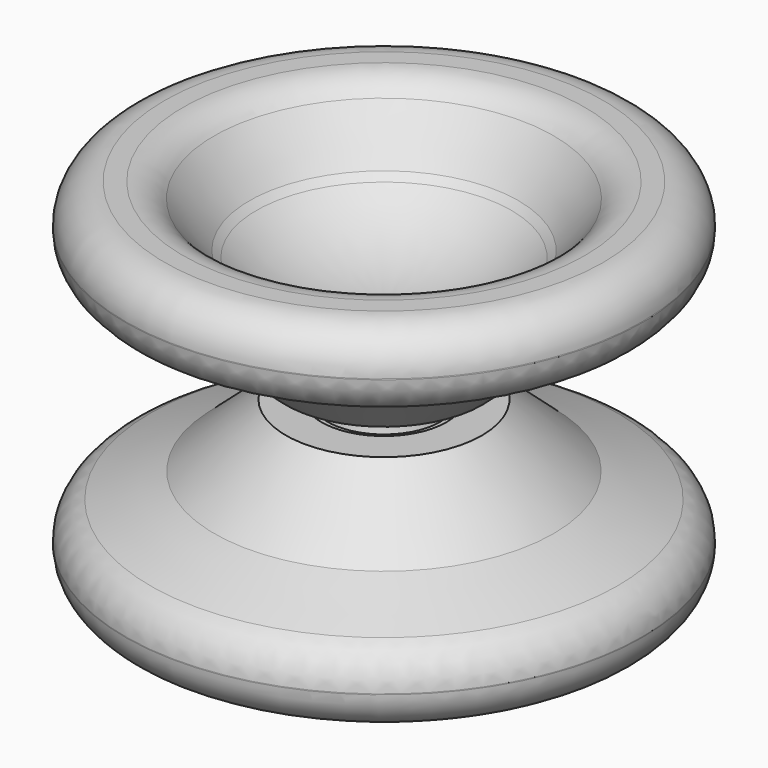
from build123d import *

# Parameters (mm, degrees)
F2_R            = 4.4
F3_R            = 20
F4_W            = 0.825
F4_H            = 3.6
F6_COPIES_COUNT = 10
F8_DEPTH        = 1.7
F8_COPIES_COUNT = 10


# Not quite as in the source:
# - a pattern or mirror of a feature is missing from the dataset's text; its kind, count and spacing are read off the source's solid


with BuildPart() as f1:
    # F0 (on Front) → F1 (revolve)
    with BuildSketch(Plane.XZ):
        Polygon((3.125, 0), (0, 0), (0, -7.5), (8.6189414508, -7.5), (15.0811627811, -13.2031436252), (20.3810585492, -20), (29, -20), (29, -12.5), (19.0302016061, -8.5869428264), (11, -1.5), (7, -1.5), (7, -2), (3.125, -2), align=None)
    revolve(axis=Axis((0, 0, -3.75), (0, 0, -1)))

    # F1_copies: F1 across plane


with BuildPart() as f1_1:
    add(f1.part)
    add(f1.part.mirror(Plane.XY))

    # F2
    f2_edges = [f1_1.edges().sort_by_distance(p)[0] for p in [
        (-29, 0, -12.5),
        (-29, 0, -20),
        (-20.381059, 0, -20),
        (-29, 0, 12.5),
        (-29, 0, 20),
        (-20.381059, 0, 20),
    ]]
    fillet(f2_edges, radius=F2_R)

    # F3
    f3_edges = [f1_1.edges().sort_by_distance(p)[0] for p in [
        (-8.618941, 0, -7.5),
        (-8.618941, 0, 7.5),
    ]]
    fillet(f3_edges, radius=F3_R)


with BuildPart() as f5:
    # F4 (on Front) → F5 (revolve)
    with BuildSketch(Plane.XZ):
        with BuildLine():
            Line((6.3, 1.7), (5.175, 1.7))
            Line((5.175, 1.7), (5.175, -1.7))
            Line((5.175, -1.7), (6.3, -1.7))
            ThreePointArc((6.3, -1.7), (6.0541289523, 0), (6.3, 1.7))
        make_face()
    revolve(axis=Axis((0, 0, -0.1984620573), (0, 0, -1)))

    # F7 (on Top) → F8 (join, symmetric)
    with BuildSketch(Plane.XY):
        with BuildLine():
            ThreePointArc((0, 4.4407169335), (0.2909, 4.8902218504), (0.6807290817, 5.2572515051))
            ThreePointArc((0.6807290817, 5.2572515051), (0, 5.3011400161), (-0.6807290817, 5.2572515051))
            ThreePointArc((-0.6807290817, 5.2572515051), (-0.2909, 4.8902218504), (0, 4.4407169335))
        make_face()
    f8 = extrude(amount=F8_DEPTH, both=True)

    # F8_copies: F8 ×10 about axis
    f8_copies_axis = Axis((0, 0, 0), (0, 0, 1))
    for i in range(1, F8_COPIES_COUNT):
        add(f8.rotate(f8_copies_axis, i * 360 / F8_COPIES_COUNT))


with BuildPart() as f6:
    # F4 (on Front) → F6 (revolve)
    with BuildSketch(Plane.XZ):
        with Locations((3.7375, 0)):
            Rectangle(F4_W, F4_H)
    revolve(axis=Axis((4.15, 0, 0), (0, 0, -1)))


with BuildPart() as f6_copies_1:
    # F6_copies: instance of F6
    add(f6.part.rotate(Axis((0, 0, 0), (0, 0, 1)), 1 * 360 / F6_COPIES_COUNT))


with BuildPart() as f6_copies_2:
    # F6_copies: instance of F6
    add(f6.part.rotate(Axis((0, 0, 0), (0, 0, 1)), 2 * 360 / F6_COPIES_COUNT))


with BuildPart() as f6_copies_3:
    # F6_copies: instance of F6
    add(f6.part.rotate(Axis((0, 0, 0), (0, 0, 1)), 3 * 360 / F6_COPIES_COUNT))


with BuildPart() as f6_copies_4:
    # F6_copies: instance of F6
    add(f6.part.rotate(Axis((0, 0, 0), (0, 0, 1)), 4 * 360 / F6_COPIES_COUNT))


with BuildPart() as f6_copies_5:
    # F6_copies: instance of F6
    add(f6.part.rotate(Axis((0, 0, 0), (0, 0, 1)), 5 * 360 / F6_COPIES_COUNT))


with BuildPart() as f6_copies_6:
    # F6_copies: instance of F6
    add(f6.part.rotate(Axis((0, 0, 0), (0, 0, 1)), 6 * 360 / F6_COPIES_COUNT))


with BuildPart() as f6_copies_7:
    # F6_copies: instance of F6
    add(f6.part.rotate(Axis((0, 0, 0), (0, 0, 1)), 7 * 360 / F6_COPIES_COUNT))


with BuildPart() as f6_copies_8:
    # F6_copies: instance of F6
    add(f6.part.rotate(Axis((0, 0, 0), (0, 0, 1)), 8 * 360 / F6_COPIES_COUNT))


with BuildPart() as f6_copies_9:
    # F6_copies: instance of F6
    add(f6.part.rotate(Axis((0, 0, 0), (0, 0, 1)), 9 * 360 / F6_COPIES_COUNT))


solid = Compound([f1_1.part, f5.part, f6.part, f6_copies_1.part, f6_copies_2.part, f6_copies_3.part, f6_copies_4.part, f6_copies_5.part, f6_copies_6.part, f6_copies_7.part, f6_copies_8.part, f6_copies_9.part])
